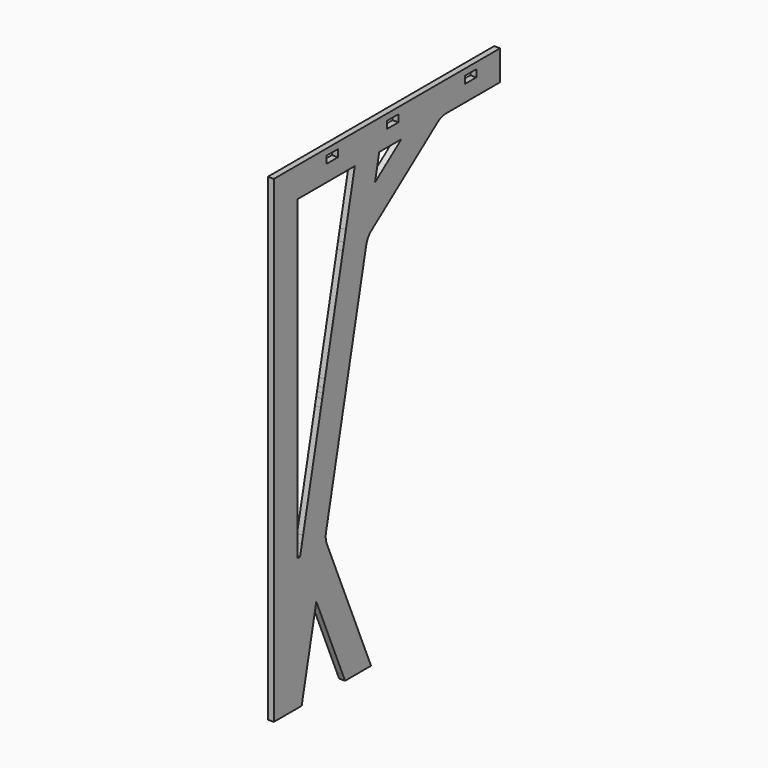
from build123d import *

# Parameters (mm, degrees)
F1_DEPTH = 2.1082
F2_R     = 0.762


# Not quite as in the source:
# - a feature names something its author has since deleted; it is built from what else it names


with BuildPart() as f1:
    # F0 (on Right) → F1 (new body)
    with BuildSketch(Plane.YZ):
        with BuildLine():
            Line((0, 169.3418), (0, 0))
            Line((0, 0), (12.335197777, 0))
            Line((12.335197777, 0), (18.8042013144, 29.896105485))
            Line((18.8042013144, 29.896105485), (30.5493542935, 2.3257501254))
            Line((30.5493542935, 2.3257501254), (31.5401391658, 0))
            Line((31.5401391658, 0), (31.5707651968, 0))
            Line((31.5707651968, 0), (40.8442968098, 0))
            Line((40.8442968098, 0), (20.5594925834, 47.616175108))
            Line((20.5594925834, 47.616175108), (39.5771112022, 135.5049402038))
            Line((39.5771112022, 135.5049402038), (73.5248959406, 160.7899383022))
            Line((73.5248959406, 160.7899383022), (100.203, 160.7899383022))
            Line((100.203, 160.7899383022), (100.203, 162.0091375))
            Line((100.203, 162.0091375), (82.1398573303, 162.0091375))
            ThreePointArc((82.1398573303, 162.0091375), (80.3438061061, 162.7530862758), (79.5998573303, 164.5491375))
            Line((79.5998573303, 164.5491375), (79.5998573303, 169.3418))
            Line((79.5998573303, 169.3418), (70.6874244764, 169.3418))
            Line((70.6874244764, 169.3418), (70.6874244764, 165.8480664454))
            Line((70.6874244764, 165.8480664454), (70.6874244764, 164.5491375))
            ThreePointArc((70.6874244764, 164.5491375), (70.0510915867, 162.8675752701), (68.4609272063, 162.0285589874))
            ThreePointArc((68.4609272063, 162.0285589874), (68.3044763435, 162.0139975214), (68.1474244764, 162.0091375))
            Line((68.1474244764, 162.0091375), (18.2118, 162.0091375))
            ThreePointArc((18.2118, 162.0091375), (16.4157487758, 162.7530862758), (15.6718, 164.5491375))
            Line((15.6718, 164.5491375), (15.6718, 169.3418))
            Line((15.6718, 169.3418), (0, 169.3418))
        make_face()
        Polygon((21.4843682503, 35.8535070154), (23.4753466245, 31.1799211209), (21.1385536773, 30.1844319338), (19.147575303, 34.8580178283), align=None, mode=Mode.SUBTRACT)
        Polygon((25.8665425285, 25.5668719827), (27.8575209028, 20.8932860882), (25.5207279555, 19.8977969011), (23.5297495813, 24.5713827956), align=None, mode=Mode.SUBTRACT)
        with BuildLine():
            Line((12.3986134924, 50.3752630702), (11.6175919588, 46.7658196656))
            Line((11.6175919588, 46.7658196656), (10.5918, 46.7658196656))
            Line((10.5918, 46.7658196656), (10.5918, 158.7579375))
            Line((10.5918, 158.7579375), (35.8507619547, 158.7579375))
            Line((35.8507619547, 158.7579375), (31.8897708968, 140.4524587956))
            Line((31.8897708968, 140.4524587956), (31.1087493632, 136.8430153909))
            Line((31.1087493632, 136.8430153909), (35.5475592049, 135.882533211))
            ThreePointArc((35.5475592049, 135.882533211), (37.1456481821, 134.7755682604), (37.4929253116, 132.8628062845))
            Line((37.4929253116, 132.8628062845), (29.5595533377, 96.1992113407))
            ThreePointArc((29.5595533377, 96.1992113407), (28.452588387, 94.6011223635), (26.5398264112, 94.2538452339))
            Line((26.5398264112, 94.2538452339), (22.1010165695, 95.2143274138))
            Line((22.1010165695, 95.2143274138), (21.7536814278, 93.6091392306))
            Line((21.7536814278, 93.6091392306), (21.4063462861, 92.0039510473))
            Line((21.4063462861, 92.0039510473), (25.8451561277, 91.0434688674))
            ThreePointArc((25.8451561277, 91.0434688674), (27.4432451049, 89.9365039168), (27.7905222345, 88.0237419409))
            Line((27.7905222345, 88.0237419409), (19.8571502605, 51.3601469971))
            ThreePointArc((19.8571502605, 51.3601469971), (18.7501853099, 49.7620580199), (16.837423334, 49.4147808903))
            Line((16.837423334, 49.4147808903), (12.3986134924, 50.3752630702))
        make_face(mode=Mode.SUBTRACT)
        Polygon((47.0613097153, 149.2568137468), (48.5785484084, 147.2197602993), (44.5044415132, 144.1852829132), (42.9872028202, 146.2223363607), align=None, mode=Mode.SUBTRACT)
        Polygon((44.8088104432, 150.074821282), (46.6876875952, 158.7579375), (56.4668125154, 158.7579375), align=None, mode=Mode.SUBTRACT)
        Polygon((63.2751536106, 161.3332132886), (64.7923923036, 159.296159841), (60.7182854085, 156.2616824549), (59.2010467154, 158.2987359025), align=None, mode=Mode.SUBTRACT)
        with BuildLine():
            Line((20.5594925834, 47.616175108), (40.8442968098, 0))
            Line((40.8442968098, 0), (43.053, 0))
            Line((43.053, 0), (23.4736756901, 45.9601445708))
            ThreePointArc((23.4736756901, 45.9601445708), (22.9941781878, 47.847708452), (23.1092917667, 49.7918185633))
            Line((23.1092917667, 49.7918185633), (40.8984089502, 132.0031391675))
            ThreePointArc((40.8984089502, 132.0031391675), (41.765080018, 134.0967787378), (43.3116785091, 135.7528217618))
            Line((43.3116785091, 135.7528217618), (72.5103326221, 157.500571119))
            ThreePointArc((72.5103326221, 157.500571119), (74.3053957564, 158.4354047741), (76.3034293547, 158.7579375))
            Line((76.3034293547, 158.7579375), (100.203, 158.7579375))
            Line((100.203, 158.7579375), (100.203, 160.7899383022))
            Line((100.203, 160.7899383022), (73.5248959406, 160.7899383022))
            Line((73.5248959406, 160.7899383022), (39.5771112022, 135.5049402038))
            Line((39.5771112022, 135.5049402038), (20.5594925834, 47.616175108))
        make_face()
        Polygon((68.1474244764, 169.3418), (18.2118, 169.3418), (18.2118, 164.5491375), (23.2918, 164.5491375), (23.2918, 167.0891375), (28.3718, 167.0891375), (28.3718, 164.5491375), (50.0948093832, 164.5491375), (50.0948093832, 167.0891375), (55.1748093832, 167.0891375), (55.1748093832, 164.5491375), (68.1474244764, 164.5491375), (68.1474244764, 165.0060867035), align=None)
        with BuildLine():
            Line((18.2118, 169.3418), (15.6718, 169.3418))
            Line((15.6718, 169.3418), (15.6718, 164.5491375))
            ThreePointArc((15.6718, 164.5491375), (16.4157487758, 162.7530862758), (18.2118, 162.0091375))
            Line((18.2118, 162.0091375), (68.1474244764, 162.0091375))
            ThreePointArc((68.1474244764, 162.0091375), (68.3044763435, 162.0139975214), (68.4609272063, 162.0285589874))
            Line((68.4609272063, 162.0285589874), (69.6856973646, 162.9407926238))
            Line((69.6856973646, 162.9407926238), (68.1474244764, 165.0060867035))
            Line((68.1474244764, 165.0060867035), (68.1474244764, 164.5491375))
            Line((68.1474244764, 164.5491375), (55.1748093832, 164.5491375))
            Line((55.1748093832, 164.5491375), (50.0948093832, 164.5491375))
            Line((50.0948093832, 164.5491375), (28.3718, 164.5491375))
            Line((28.3718, 164.5491375), (23.2918, 164.5491375))
            Line((23.2918, 164.5491375), (18.2118, 164.5491375))
            Line((18.2118, 164.5491375), (18.2118, 169.3418))
        make_face()
        Polygon((20.8691658762, 89.5214045307), (12.9357939022, 52.8578095868), (17.3746037439, 51.8973274069), (18.6675621562, 57.872655888), (16.1850156395, 58.4098362979), (17.2593764593, 63.3749293312), (19.7419229759, 62.8377489213), (22.9432277355, 77.6323837102), (20.4606812189, 78.16956412), (21.5350420386, 83.1346571533), (24.0175885553, 82.5974767434), (25.3079757178, 88.5609223508), align=None)
        Polygon((35.010378795, 133.3999866944), (30.5715689534, 134.3604688743), (22.6381969794, 97.6968739305), (27.077006821, 96.7363917505), (28.3673939836, 102.6998373579), (25.884847467, 103.2370177677), (26.9592082867, 108.202110801), (29.4417548033, 107.6649303911), (32.643059563, 122.45956518), (30.1605130463, 122.9967455899), (31.2348738661, 127.9618386231), (33.7174203827, 127.4246582133), align=None)
        with BuildLine():
            Line((12.9357939022, 52.8578095868), (12.3986134924, 50.3752630702))
            Line((12.3986134924, 50.3752630702), (16.837423334, 49.4147808903))
            ThreePointArc((16.837423334, 49.4147808903), (18.7501853099, 49.7620580199), (19.8571502605, 51.3601469971))
            Line((19.8571502605, 51.3601469971), (27.7905222345, 88.0237419409))
            ThreePointArc((27.7905222345, 88.0237419409), (27.4432451049, 89.9365039168), (25.8451561277, 91.0434688674))
            Line((25.8451561277, 91.0434688674), (21.4063462861, 92.0039510473))
            Line((21.4063462861, 92.0039510473), (20.8691658762, 89.5214045307))
            Line((20.8691658762, 89.5214045307), (25.3079757178, 88.5609223508))
            Line((25.3079757178, 88.5609223508), (24.0175885553, 82.5974767434))
            Line((24.0175885553, 82.5974767434), (22.9432277355, 77.6323837102))
            Line((22.9432277355, 77.6323837102), (19.7419229759, 62.8377489213))
            Line((19.7419229759, 62.8377489213), (18.6675621562, 57.872655888))
            Line((18.6675621562, 57.872655888), (17.3746037439, 51.8973274069))
            Line((17.3746037439, 51.8973274069), (12.9357939022, 52.8578095868))
        make_face()
        with BuildLine():
            Line((35.5475592049, 135.882533211), (31.1087493632, 136.8430153909))
            Line((31.1087493632, 136.8430153909), (30.5715689534, 134.3604688743))
            Line((30.5715689534, 134.3604688743), (35.010378795, 133.3999866944))
            Line((35.010378795, 133.3999866944), (33.7174203827, 127.4246582133))
            Line((33.7174203827, 127.4246582133), (32.643059563, 122.45956518))
            Line((32.643059563, 122.45956518), (29.4417548033, 107.6649303911))
            Line((29.4417548033, 107.6649303911), (28.3673939836, 102.6998373579))
            Line((28.3673939836, 102.6998373579), (27.077006821, 96.7363917505))
            Line((27.077006821, 96.7363917505), (22.6381969794, 97.6968739305))
            Line((22.6381969794, 97.6968739305), (22.1010165695, 95.2143274138))
            Line((22.1010165695, 95.2143274138), (26.5398264112, 94.2538452339))
            ThreePointArc((26.5398264112, 94.2538452339), (28.452588387, 94.6011223635), (29.5595533377, 96.1992113407))
            Line((29.5595533377, 96.1992113407), (37.4929253116, 132.8628062845))
            ThreePointArc((37.4929253116, 132.8628062845), (37.1456481821, 134.7755682604), (35.5475592049, 135.882533211))
        make_face()
        Polygon((100.203, 169.3418), (82.1398573303, 169.3418), (82.1398573303, 164.5491375), (84.5702663064, 164.5491375), (84.5702663064, 167.0891375), (89.6502663064, 167.0891375), (89.6502663064, 164.5491375), (100.203, 164.5491375), align=None)
        with BuildLine():
            Line((82.1398573303, 169.3418), (79.5998573303, 169.3418))
            Line((79.5998573303, 169.3418), (79.5998573303, 164.5491375))
            ThreePointArc((79.5998573303, 164.5491375), (80.3438061061, 162.7530862758), (82.1398573303, 162.0091375))
            Line((82.1398573303, 162.0091375), (100.203, 162.0091375))
            Line((100.203, 162.0091375), (100.203, 164.5491375))
            Line((100.203, 164.5491375), (89.6502663064, 164.5491375))
            Line((89.6502663064, 164.5491375), (84.5702663064, 164.5491375))
            Line((84.5702663064, 164.5491375), (82.1398573303, 164.5491375))
            Line((82.1398573303, 164.5491375), (82.1398573303, 169.3418))
        make_face()
        with BuildLine():
            Line((70.6874244764, 169.3418), (68.1474244764, 169.3418))
            Line((68.1474244764, 169.3418), (68.1474244764, 165.0060867035))
            Line((68.1474244764, 165.0060867035), (69.6856973646, 162.9407926238))
            Line((69.6856973646, 162.9407926238), (68.4609272063, 162.0285589874))
            ThreePointArc((68.4609272063, 162.0285589874), (70.0510915867, 162.8675752701), (70.6874244764, 164.5491375))
            Line((70.6874244764, 164.5491375), (70.6874244764, 165.8480664454))
            Line((70.6874244764, 165.8480664454), (70.6874244764, 169.3418))
        make_face()
        Polygon((21.1385536773, 30.1844319338), (23.4753466245, 31.1799211209), (21.4843682503, 35.8535070154), (19.147575303, 34.8580178283), align=None)
        Polygon((25.5207279555, 19.8977969011), (27.8575209028, 20.8932860882), (25.8665425285, 25.5668719827), (23.5297495813, 24.5713827956), align=None)
        Polygon((44.5044415132, 144.1852829132), (48.5785484084, 147.2197602993), (47.0613097153, 149.2568137468), (42.9872028202, 146.2223363607), align=None)
        Polygon((60.7182854085, 156.2616824549), (64.7923923036, 159.296159841), (63.2751536106, 161.3332132886), (59.2010467154, 158.2987359025), align=None)
        Polygon((16.1850156395, 58.4098362979), (18.6675621562, 57.872655888), (19.7419229759, 62.8377489213), (17.2593764593, 63.3749293312), align=None)
        Polygon((22.9432277355, 77.6323837102), (24.0175885553, 82.5974767434), (21.5350420386, 83.1346571533), (20.4606812189, 78.16956412), align=None)
        Polygon((32.643059563, 122.45956518), (33.7174203827, 127.4246582133), (31.2348738661, 127.9618386231), (30.1605130463, 122.9967455899), align=None)
        Polygon((25.884847467, 103.2370177677), (28.3673939836, 102.6998373579), (29.4417548033, 107.6649303911), (26.9592082867, 108.202110801), align=None)
    extrude(amount=F1_DEPTH)

    # F2
    f2_edges = [f1.edges().sort_by_distance(p)[0] for p in [
        (0, 32.00385, 90.897479),
        (0, 33.263338, 22.980072),
        (0, 22.994178, 47.847708),
        (0, 41.76508, 134.096779),
        (0, 57.911006, 146.626696),
        (0, 74.305396, 158.435405),
        (0, 88.253215, 158.757937),
    ]]
    fillet(f2_edges, radius=F2_R)


solid = f1.part
